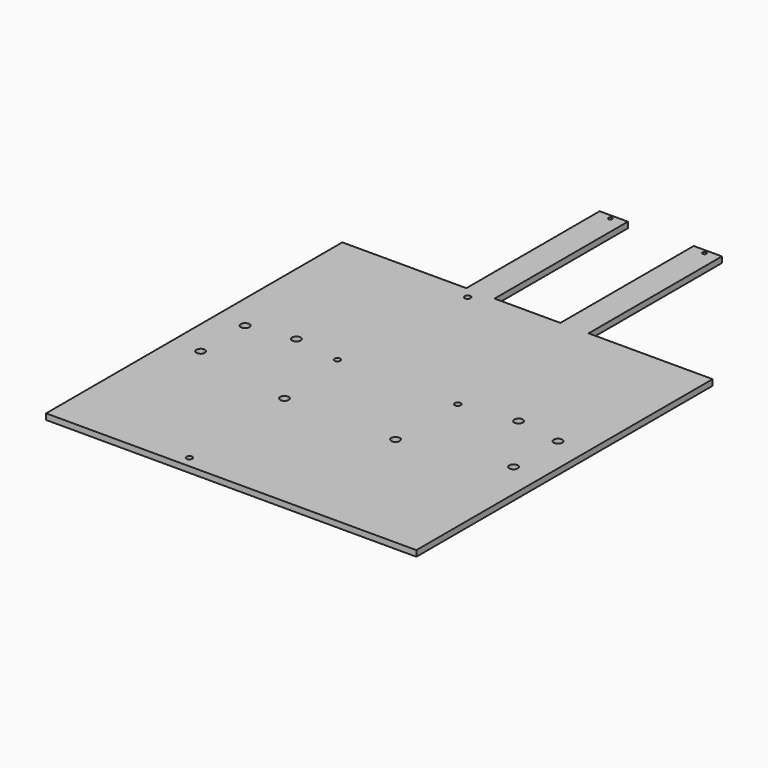
from build123d import *

# Parameters (mm, degrees)
F0_W     = 51.8
F0_H     = 10
F0_W_2   = 15.24
F0_H_2   = 34.925
F0_R     = 2.3114
F0_R_2   = 1.05
F0_R_3   = 1.5875
F0_W_3   = 9.38
F1_DEPTH = 3.175
F2_DEPTH = 90


# Not quite as in the source:
# - a length typed as a fraction of an inch, garbled in the dataset ("3 / 203.2 mm" for 3/8 in), is restored
# - a feature names something its author has since deleted; it is built from what else it names


with BuildPart() as f1:
    # F0 (on Top) → F1 (new body)
    with BuildSketch(Plane.XY):
        Polygon((42.4, -100), (100, -100), (100, -75.075), (48.2, -75.075), (48.2, -65.075), (33.02, -65.075), (33.02, -100), align=None)
        with Locations((74.1, -70.075)):
            Rectangle(F0_W, F0_H)
        Polygon((33.02, -140), (33.02, -100), (17.78, -100), (17.78, -140), (17.78, -190), (25.4, -190), (33.02, -190), align=None)
        with BuildLine():
            ThreePointArc((26.45, -187.7), (26.1424621202, -188.4424621202), (25.4, -188.75))
            ThreePointArc((25.4, -188.75), (24.6575378798, -186.9575378798), (26.45, -187.7))
        make_face(mode=Mode.SUBTRACT)
        with Locations((25.4, -82.5375)):
            Rectangle(F0_W_2, F0_H_2)
        with Locations((74.1, -60.075)):
            Rectangle(F0_W, F0_H)
        Polygon((0, -100), (17.78, -100), (17.78, -65.075), (-17.78, -65.075), (-17.78, -100), align=None)
        Polygon((17.78, -65.075), (33.02, -65.075), (48.2, -65.075), (48.2, -55.075), (-48.2, -55.075), (-48.2, -65.075), (-33.02, -65.075), (-17.78, -65.075), align=None)
        with BuildLine():
            Line((48.2, -55.075), (100, -55.075))
            Line((100, -55.075), (100, -26.575))
            Line((100, -26.575), (32.3114, -26.575))
            ThreePointArc((32.3114, -26.575), (30, -28.8864), (27.6886, -26.575))
            Line((27.6886, -26.575), (0, -26.575))
            Line((0, -26.575), (-27.6886, -26.575))
            ThreePointArc((-27.6886, -26.575), (-30, -28.8864), (-32.3114, -26.575))
            Line((-32.3114, -26.575), (-100, -26.575))
            Line((-100, -26.575), (-100, -55.075))
            Line((-100, -55.075), (-48.2, -55.075))
            Line((-48.2, -55.075), (48.2, -55.075))
        make_face()
        with BuildLine():
            Line((32.3114, -26.575), (100, -26.575))
            Line((100, -26.575), (100, 0))
            Line((100, 0), (0, 0))
            Line((0, 0), (0, -10.4469014332))
            Line((0, -10.4469014332), (0, -26.575))
            Line((0, -26.575), (27.6886, -26.575))
            ThreePointArc((27.6886, -26.575), (30, -24.2636), (32.3114, -26.575))
        make_face()
        with Locations((84.5, -15)):
            Circle(F0_R, mode=Mode.SUBTRACT)
        Polygon((-17.78, -140), (-17.78, -100), (-27.462, -100), (-33.02, -100), (-33.02, -140), (-33.02, -190), (-25.4, -190), (-17.78, -190), align=None)
        with BuildLine():
            ThreePointArc((-24.35, -187.7), (-24.6575378798, -188.4424621202), (-25.4, -188.75))
            ThreePointArc((-25.4, -188.75), (-26.1424621202, -186.9575378798), (-24.35, -187.7))
        make_face(mode=Mode.SUBTRACT)
        with Locations((-25.4, -137.7)):
            Circle(F0_R_2, mode=Mode.SUBTRACT)
        Polygon((-27.462, -100), (-17.78, -100), (-17.78, -65.075), (-33.02, -65.075), (-33.02, -100), align=None)
        with BuildLine():
            ThreePointArc((-25.8745, -93.912), (-26.3394679849, -95.0345320151), (-27.462, -95.4995))
            ThreePointArc((-27.462, -95.4995), (-29.0495, -93.912), (-27.462, -92.3245))
            ThreePointArc((-27.462, -92.3245), (-26.3394679849, -92.7894679849), (-25.8745, -93.912))
        make_face(mode=Mode.SUBTRACT)
        with BuildLine():
            Line((0, 0), (100, 0))
            Line((100, 0), (100, 55.075))
            Line((100, 55.075), (48.2, 55.075))
            Line((48.2, 55.075), (48.2, 65.075))
            Line((48.2, 65.075), (42.4, 65.075))
            Line((42.4, 65.075), (42.4, 18.9709383994))
            Line((42.4, 18.9709383994), (42.4, 9.75))
            Line((42.4, 9.75), (30.355, 9.75))
            Line((30.355, 9.75), (-42.4, 9.75))
            Line((-42.4, 9.75), (-42.4, 65.075))
            Line((-42.4, 65.075), (-48.2, 65.075))
            Line((-48.2, 65.075), (-48.2, 55.075))
            Line((-48.2, 55.075), (-100, 55.075))
            Line((-100, 55.075), (-100, 0))
            Line((-100, 0), (-100, -26.575))
            Line((-100, -26.575), (-32.3114, -26.575))
            ThreePointArc((-32.3114, -26.575), (-30, -24.2636), (-27.6886, -26.575))
            Line((-27.6886, -26.575), (0, -26.575))
            Line((0, -26.575), (0, -10.4469014332))
            Line((0, -10.4469014332), (0, 0))
        make_face()
        with BuildLine():
            ThreePointArc((-82.1886, -15), (-86.134406614, -16.634406614), (-84.5, -12.6886))
            ThreePointArc((-84.5, -12.6886), (-82.865593386, -13.365593386), (-82.1886, -15))
        make_face(mode=Mode.SUBTRACT)
        with BuildLine():
            ThreePointArc((-82.1886, 15), (-82.865593386, 13.365593386), (-84.5, 12.6886))
            ThreePointArc((-84.5, 12.6886), (-86.134406614, 16.634406614), (-82.1886, 15))
        make_face(mode=Mode.SUBTRACT)
        with Locations((-60, 18.9709383994)):
            Circle(F0_R, mode=Mode.SUBTRACT)
        with BuildLine():
            ThreePointArc((62.3114, 18.9709383994), (60, 16.6595383994), (57.6886, 18.9709383994))
            ThreePointArc((57.6886, 18.9709383994), (60, 21.2823383994), (62.3114, 18.9709383994))
        make_face(mode=Mode.SUBTRACT)
        with Locations((84.5, 15)):
            Circle(F0_R, mode=Mode.SUBTRACT)
        with Locations((-74.1, -60.075)):
            Rectangle(F0_W, F0_H)
        Polygon((-33.02, -100), (-33.02, -65.075), (-48.2, -65.075), (-48.2, -75.075), (-100, -75.075), (-100, -100), (-42.4, -100), align=None)
        with Locations((74.1, 60.075)):
            Rectangle(F0_W, F0_H)
        with Locations((-74.1, -70.075)):
            Rectangle(F0_W, F0_H)
        with Locations((74.1, 70.075)):
            Rectangle(F0_W, F0_H)
        Polygon((48.2, 75.075), (100, 75.075), (100, 100), (42.4, 100), (42.4, 65.075), (48.2, 65.075), align=None)
        Polygon((42.4, 18.9709383994), (42.4, 65.075), (42.4, 100), (33.02, 100), (17.78, 100), (0, 100), (-17.78, 100), (-27.462, 100), (-33.02, 100), (-33.02, 65.075), (-42.4, 65.075), (-42.4, 9.75), (30.355, 9.75), (42.4, 9.75), align=None)
        with Locations((-34.645, 14.954)):
            Circle(F0_R_3, mode=Mode.SUBTRACT)
        with BuildLine():
            ThreePointArc((-27.462, 92.3245), (-29.0495, 93.912), (-27.462, 95.4995))
            ThreePointArc((-27.462, 95.4995), (-26.3394679849, 95.0345320151), (-25.8745, 93.912))
            ThreePointArc((-25.8745, 93.912), (-26.3394679849, 92.7894679849), (-27.462, 92.3245))
        make_face(mode=Mode.SUBTRACT)
        with BuildLine():
            ThreePointArc((31.9425, 14.954), (31.4775320151, 13.8314679849), (30.355, 13.3665))
            ThreePointArc((30.355, 13.3665), (29.2324679849, 13.8314679849), (28.7675, 14.954))
            ThreePointArc((28.7675, 14.954), (30.355, 16.5415), (31.9425, 14.954))
        make_face(mode=Mode.SUBTRACT)
        with Locations((-74.1, 60.075)):
            Rectangle(F0_W, F0_H)
        with Locations((-74.1, 70.075)):
            Rectangle(F0_W, F0_H)
        Polygon((17.78, 100), (33.02, 100), (33.02, 140), (33.02, 190), (25.4, 190), (17.78, 190), (17.78, 140), align=None)
        with BuildLine():
            ThreePointArc((26.45, 187.7), (24.6575378798, 186.9575378798), (25.4, 188.75))
            ThreePointArc((25.4, 188.75), (26.1424621202, 188.4424621202), (26.45, 187.7))
        make_face(mode=Mode.SUBTRACT)
        Polygon((-100, 100), (-100, 75.075), (-48.2, 75.075), (-48.2, 65.075), (-42.4, 65.075), (-42.4, 100), align=None)
        with Locations((-37.71, 82.5375)):
            Rectangle(F0_W_3, F0_H_2)
        Polygon((-27.462, 100), (-17.78, 100), (-17.78, 140), (-17.78, 190), (-25.4, 190), (-33.02, 190), (-33.02, 140), (-33.02, 100), align=None)
        with BuildLine():
            ThreePointArc((-24.35, 187.7), (-26.1424621202, 186.9575378798), (-25.4, 188.75))
            ThreePointArc((-25.4, 188.75), (-24.6575378798, 188.4424621202), (-24.35, 187.7))
        make_face(mode=Mode.SUBTRACT)
        with Locations((-25.4, -137.7)):
            Circle(F0_R_2)
    extrude(amount=F1_DEPTH)

    # F2 (cut): faces of the model
    f2_faces = [f1.faces().sort_by_distance(p)[0] for p in [
        (25.4, -190, 1.5875),
        (-25.4, -190, 1.5875),
    ]]
    extrude(f2_faces, amount=-F2_DEPTH, mode=Mode.SUBTRACT)


solid = f1.part
